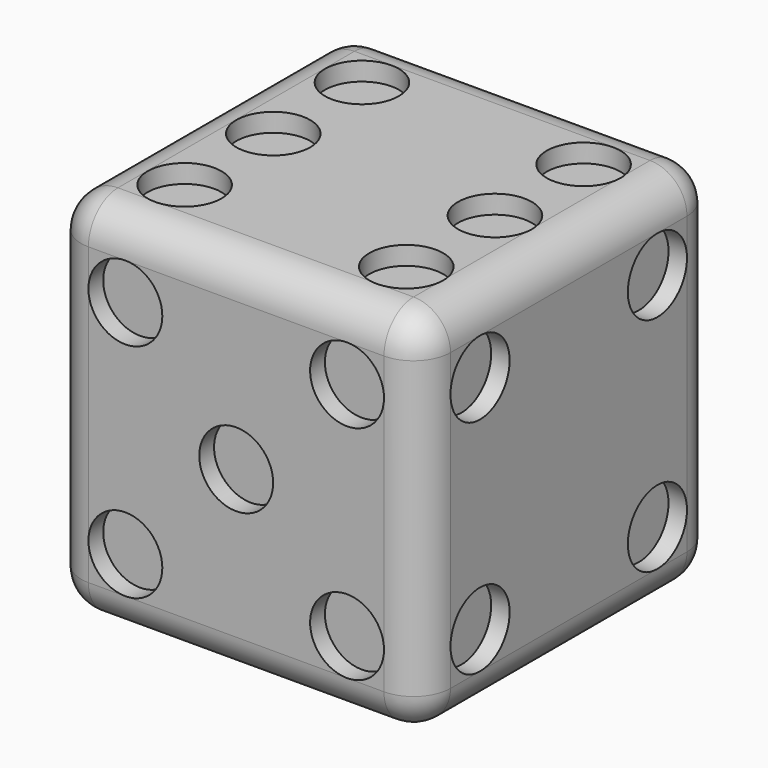
from build123d import *

# Parameters (mm, degrees)
F0_W          = 20
F0_H          = 20
F1_DEPTH      = 20
F3_R          = 2
F8_DEPTH      = 1
F2_R          = 2
F11_DEPTH     = 1
F6_R          = 2.787917168
F12_DEPTH     = 1
F4_R          = 2
F13_DEPTH     = 1
F14_DEPTH     = 1
F5_R          = 2
F15_DEPTH     = 1
F7_R          = 2
F16_DEPTH     = 1
F17_T1_DEPTH  = 16
F17_T3_DEPTH  = 16
F17_T5_DEPTH  = 16
F17_S9_W      = 2
F17_S9_H      = 2
F17_T10_DEPTH = 2
F17_S15_W     = 2
F17_S15_H     = 2
F17_T16_DEPTH = 2
F17_S21_W     = 2
F17_S21_H     = 2
F17_T22_DEPTH = 2
F17_S27_W     = 2
F17_S27_H     = 2
F17_T28_DEPTH = 2
F17_S33_W     = 2
F17_S33_H     = 2
F17_T34_DEPTH = 2
F17_S39_W     = 2
F17_S39_H     = 2
F17_T40_DEPTH = 2
F17_S45_W     = 2
F17_S45_H     = 2
F17_T46_DEPTH = 2
F17_S51_W     = 2
F17_S51_H     = 2
F17_T52_DEPTH = 2


# Not quite as in the source:
# - a fillet or chamfer that OpenCascade refuses, or shapes differently, is made with other operations: its cross-section is extruded or revolved along the edge and cut away or added
# - a feature of the source that left no trace in its solid (it failed there, or was rolled back) is left out


with BuildPart() as f1:
    # F0 (on Top) → F1 (new body)
    with BuildSketch(Plane.XY):
        with Locations((10, 10)):
            Rectangle(F0_W, F0_H)
    extrude(amount=F1_DEPTH)

    # F3 (on face) → F8 (cut)
    with BuildSketch(Plane.XY.offset(20)):
        with Locations((4.0282921307, 15.9717078693)):
            Circle(F3_R)
        with Locations((4.0282921307, 9.9717078693)):
            Circle(F3_R)
        with Locations((4.0282921307, 3.9717078693)):
            Circle(F3_R)
        with Locations((16.0282921307, 15.9717078693)):
            Circle(F3_R)
        with Locations((16.0282921307, 9.9717078693)):
            Circle(F3_R)
        with Locations((16.0282921307, 3.9717078693)):
            Circle(F3_R)
    extrude(amount=-F8_DEPTH, mode=Mode.SUBTRACT)

    # F2 (on Top) → F11 (cut)
    with BuildSketch(Plane.XY):
        with Locations((10, 10)):
            Circle(F2_R)
    extrude(amount=F11_DEPTH, mode=Mode.SUBTRACT)

    # F6 (on face) → F12 (cut)
    with BuildSketch(Plane(origin=(0, 0, 0), x_dir=(0, -1, 0), z_dir=(-1, 0, 0))):
        with Locations((-15.4005342424, 15.4005342424)):
            Circle(F6_R)
        with Locations((-10.667038206, 10.667038206)):
            Circle(F6_R)
        with Locations((-5.3520903582, 5.3520903582)):
            Circle(F6_R)
    extrude(amount=-F12_DEPTH, mode=Mode.SUBTRACT)

    # F4 (on Front) → F13 (cut)
    with BuildSketch(Plane.XZ):
        with Locations((16, 4)):
            Circle(F4_R)
        with Locations((4, 16)):
            Circle(F4_R)
        with Locations((16, 16)):
            Circle(F4_R)
        with Locations((4, 4)):
            Circle(F4_R)
        with Locations((10, 10)):
            Circle(F4_R)
    extrude(amount=-F13_DEPTH, mode=Mode.SUBTRACT)

    # F6 (on face) → F14 (cut)
    with BuildSketch(Plane(origin=(0, 0, 0), x_dir=(0, -1, 0), z_dir=(-1, 0, 0))):
        with Locations((-15.4005342424, 15.4005342424)):
            Circle(F6_R)
        with Locations((-10.667038206, 10.667038206)):
            Circle(F6_R)
        with Locations((-5.3520903582, 5.3520903582)):
            Circle(F6_R)
    extrude(amount=-F14_DEPTH, mode=Mode.SUBTRACT)

    # F5 (on face) → F15 (cut)
    with BuildSketch(Plane(origin=(0, 20, 0), x_dir=(-1, 0, 0), z_dir=(0, 1, 0))):
        with Locations((-13.3333333333, 13.3333333333)):
            Circle(F5_R)
        with Locations((-6.6666666667, 6.6666666667)):
            Circle(F5_R)
    extrude(amount=-F15_DEPTH, mode=Mode.SUBTRACT)

    # F7 (on face) → F16 (cut)
    with BuildSketch(Plane.YZ.offset(20)):
        with Locations((16, 4)):
            Circle(F7_R)
        with Locations((16, 16)):
            Circle(F7_R)
        with Locations((4, 16)):
            Circle(F7_R)
        with Locations((4, 4)):
            Circle(F7_R)
    extrude(amount=-F16_DEPTH, mode=Mode.SUBTRACT)

    # F17: fillet of radius 2 on 12 edges, made by hand

    # F17_s2 → F17_t1 (cut)
    with BuildSketch(Plane.YZ.offset(2)):
        with BuildLine():
            ThreePointArc((20, 2), (19.4142135624, 0.5857864376), (18, 0))
            Line((18, 0), (20, 0))
            Line((20, 0), (20, 2))
        make_face()
        with BuildLine():
            ThreePointArc((2, 0), (0.5857864376, 0.5857864376), (0, 2))
            Line((0, 2), (0, 0))
            Line((0, 0), (2, 0))
        make_face()
        with BuildLine():
            ThreePointArc((2, 20), (0.5857864376, 19.4142135624), (0, 18))
            Line((0, 18), (0, 20))
            Line((0, 20), (2, 20))
        make_face()
        with BuildLine():
            ThreePointArc((20, 18), (19.4142135624, 19.4142135624), (18, 20))
            Line((18, 20), (20, 20))
            Line((20, 20), (20, 18))
        make_face()
    extrude(amount=F17_T1_DEPTH, mode=Mode.SUBTRACT)

    # F17_s4 → F17_t3 (cut)
    with BuildSketch(Plane.XZ.offset(-18)):
        with BuildLine():
            ThreePointArc((18, 0), (19.4142135624, 0.5857864376), (20, 2))
            Line((20, 2), (20, 0))
            Line((20, 0), (18, 0))
        make_face()
        with BuildLine():
            ThreePointArc((0, 2), (0.5857864376, 0.5857864376), (2, 0))
            Line((2, 0), (0, 0))
            Line((0, 0), (0, 2))
        make_face()
        with BuildLine():
            ThreePointArc((0, 18), (0.5857864376, 19.4142135624), (2, 20))
            Line((2, 20), (0, 20))
            Line((0, 20), (0, 18))
        make_face()
        with BuildLine():
            ThreePointArc((18, 20), (19.4142135624, 19.4142135624), (20, 18))
            Line((20, 18), (20, 20))
            Line((20, 20), (18, 20))
        make_face()
    extrude(amount=F17_T3_DEPTH, mode=Mode.SUBTRACT)

    # F17_s6 → F17_t5 (cut)
    with BuildSketch(Plane.XY.offset(2)):
        with BuildLine():
            ThreePointArc((0, 2), (0.5857864376, 0.5857864376), (2, 0))
            Line((2, 0), (0, 0))
            Line((0, 0), (0, 2))
        make_face()
        with BuildLine():
            ThreePointArc((0, 18), (0.5857864376, 19.4142135624), (2, 20))
            Line((2, 20), (0, 20))
            Line((0, 20), (0, 18))
        make_face()
        with BuildLine():
            ThreePointArc((18, 0), (19.4142135624, 0.5857864376), (20, 2))
            Line((20, 2), (20, 0))
            Line((20, 0), (18, 0))
        make_face()
        with BuildLine():
            ThreePointArc((18, 20), (19.4142135624, 19.4142135624), (20, 18))
            Line((20, 18), (20, 20))
            Line((20, 20), (18, 20))
        make_face()
    extrude(amount=F17_T5_DEPTH, mode=Mode.SUBTRACT)


with BuildPart() as f17_tool8:
    # F17_s9 → F17_t10 (new body)
    with BuildSketch(Plane.YZ.offset(18)):
        with Locations((19, 1)):
            Rectangle(F17_S9_W, F17_S9_H)
    extrude(amount=F17_T10_DEPTH)

    # F17_s11 → F17_t12 (revolve, cut)
    with BuildSketch(Plane(origin=(18, 18, 2), x_dir=(0, -0.7071067812, 0.7071067812), z_dir=(0, 0.7071067812, 0.7071067812))):
        with BuildLine():
            ThreePointArc((0, -2), (2, 0), (0, 2))
            Line((0, 2), (0, -2))
        make_face()
    revolve(axis=Axis((18, 18, 2), (1, 0, 0)), mode=Mode.SUBTRACT)


with BuildPart() as f1_1:
    add(f1.part)

    # F17_t7: cut F17_tool8
    add(f17_tool8.part, mode=Mode.SUBTRACT)


with BuildPart() as f17_tool14:
    # F17_s15 → F17_t16 (new body)
    with BuildSketch(Plane.YZ.offset(2)):
        with Locations((19, 1)):
            Rectangle(F17_S15_W, F17_S15_H)
    extrude(amount=-F17_T16_DEPTH)

    # F17_s17 → F17_t18 (revolve, cut)
    with BuildSketch(Plane(origin=(2, 18, 2), x_dir=(0, -0.7071067812, 0.7071067812), z_dir=(0, -0.7071067812, -0.7071067812))):
        with BuildLine():
            ThreePointArc((0, -2), (2, 0), (0, 2))
            Line((0, 2), (0, -2))
        make_face()
    revolve(axis=Axis((2, 18, 2), (-1, 0, 0)), mode=Mode.SUBTRACT)


with BuildPart() as f1_2:
    add(f1_1.part)

    # F17_t13: cut F17_tool14
    add(f17_tool14.part, mode=Mode.SUBTRACT)


with BuildPart() as f17_tool20:
    # F17_s21 → F17_t22 (new body)
    with BuildSketch(Plane.YZ.offset(18)):
        with Locations((1, 1)):
            Rectangle(F17_S21_W, F17_S21_H)
    extrude(amount=F17_T22_DEPTH)

    # F17_s23 → F17_t24 (revolve, cut)
    with BuildSketch(Plane(origin=(18, 2, 2), x_dir=(0, 0.7071067812, 0.7071067812), z_dir=(0, 0.7071067812, -0.7071067812))):
        with BuildLine():
            ThreePointArc((0, -2), (2, 0), (0, 2))
            Line((0, 2), (0, -2))
        make_face()
    revolve(axis=Axis((18, 2, 2), (1, 0, 0)), mode=Mode.SUBTRACT)


with BuildPart() as f1_3:
    add(f1_2.part)

    # F17_t19: cut F17_tool20
    add(f17_tool20.part, mode=Mode.SUBTRACT)


with BuildPart() as f17_tool26:
    # F17_s27 → F17_t28 (new body)
    with BuildSketch(Plane.YZ.offset(2)):
        with Locations((1, 1)):
            Rectangle(F17_S27_W, F17_S27_H)
    extrude(amount=-F17_T28_DEPTH)

    # F17_s29 → F17_t30 (revolve, cut)
    with BuildSketch(Plane(origin=(2, 2, 2), x_dir=(0, 0.7071067812, 0.7071067812), z_dir=(0, -0.7071067812, 0.7071067812))):
        with BuildLine():
            ThreePointArc((0, -2), (2, 0), (0, 2))
            Line((0, 2), (0, -2))
        make_face()
    revolve(axis=Axis((2, 2, 2), (-1, 0, 0)), mode=Mode.SUBTRACT)


with BuildPart() as f1_4:
    add(f1_3.part)

    # F17_t25: cut F17_tool26
    add(f17_tool26.part, mode=Mode.SUBTRACT)


with BuildPart() as f17_tool32:
    # F17_s33 → F17_t34 (new body)
    with BuildSketch(Plane.YZ.offset(2)):
        with Locations((1, 19)):
            Rectangle(F17_S33_W, F17_S33_H)
    extrude(amount=-F17_T34_DEPTH)

    # F17_s35 → F17_t36 (revolve, cut)
    with BuildSketch(Plane(origin=(2, 2, 18), x_dir=(0, 0.7071067812, -0.7071067812), z_dir=(0, 0.7071067812, 0.7071067812))):
        with BuildLine():
            ThreePointArc((0, -2), (2, 0), (0, 2))
            Line((0, 2), (0, -2))
        make_face()
    revolve(axis=Axis((2, 2, 18), (-1, 0, 0)), mode=Mode.SUBTRACT)


with BuildPart() as f1_5:
    add(f1_4.part)

    # F17_t31: cut F17_tool32
    add(f17_tool32.part, mode=Mode.SUBTRACT)


with BuildPart() as f17_tool38:
    # F17_s39 → F17_t40 (new body)
    with BuildSketch(Plane.YZ.offset(2)):
        with Locations((19, 19)):
            Rectangle(F17_S39_W, F17_S39_H)
    extrude(amount=-F17_T40_DEPTH)

    # F17_s41 → F17_t42 (revolve, cut)
    with BuildSketch(Plane(origin=(2, 18, 18), x_dir=(0, -0.7071067812, -0.7071067812), z_dir=(0, 0.7071067812, -0.7071067812))):
        with BuildLine():
            ThreePointArc((0, -2), (2, 0), (0, 2))
            Line((0, 2), (0, -2))
        make_face()
    revolve(axis=Axis((2, 18, 18), (-1, 0, 0)), mode=Mode.SUBTRACT)


with BuildPart() as f1_6:
    add(f1_5.part)

    # F17_t37: cut F17_tool38
    add(f17_tool38.part, mode=Mode.SUBTRACT)


with BuildPart() as f17_tool44:
    # F17_s45 → F17_t46 (new body)
    with BuildSketch(Plane.YZ.offset(18)):
        with Locations((1, 19)):
            Rectangle(F17_S45_W, F17_S45_H)
    extrude(amount=F17_T46_DEPTH)

    # F17_s47 → F17_t48 (revolve, cut)
    with BuildSketch(Plane(origin=(18, 2, 18), x_dir=(0, 0.7071067812, -0.7071067812), z_dir=(0, -0.7071067812, -0.7071067812))):
        with BuildLine():
            ThreePointArc((0, -2), (2, 0), (0, 2))
            Line((0, 2), (0, -2))
        make_face()
    revolve(axis=Axis((18, 2, 18), (1, 0, 0)), mode=Mode.SUBTRACT)


with BuildPart() as f1_7:
    add(f1_6.part)

    # F17_t43: cut F17_tool44
    add(f17_tool44.part, mode=Mode.SUBTRACT)


with BuildPart() as f17_tool50:
    # F17_s51 → F17_t52 (new body)
    with BuildSketch(Plane.YZ.offset(18)):
        with Locations((19, 19)):
            Rectangle(F17_S51_W, F17_S51_H)
    extrude(amount=F17_T52_DEPTH)

    # F17_s53 → F17_t54 (revolve, cut)
    with BuildSketch(Plane(origin=(18, 18, 18), x_dir=(0, -0.7071067812, -0.7071067812), z_dir=(0, -0.7071067812, 0.7071067812))):
        with BuildLine():
            ThreePointArc((0, -2), (2, 0), (0, 2))
            Line((0, 2), (0, -2))
        make_face()
    revolve(axis=Axis((18, 18, 18), (1, 0, 0)), mode=Mode.SUBTRACT)


with BuildPart() as f1_8:
    add(f1_7.part)

    # F17_t49: cut F17_tool50
    add(f17_tool50.part, mode=Mode.SUBTRACT)


solid = f1_8.part
